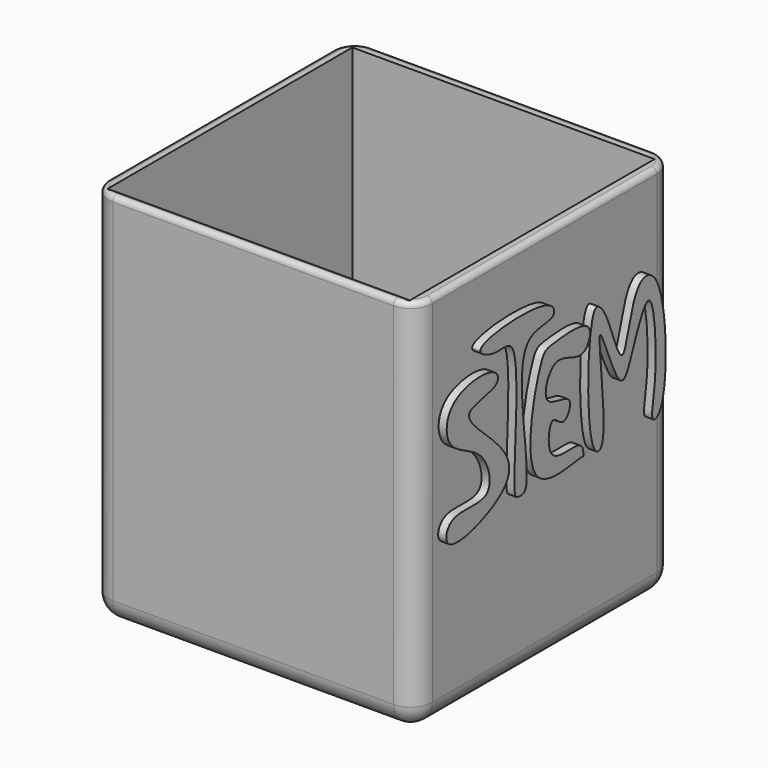
from build123d import *

# Parameters (mm, degrees)
F0_W        = 76.2
F0_H        = 76.2
F1_DEPTH    = 88.9
F2_T        = -2.54
F3_R        = 5.08
F4_R        = 1.27
F5_T1_DEPTH = 71.12
F6_R        = 5.08
F8_DEPTH    = 1.905
F10_DEPTH   = 1.905
F12_DEPTH   = 1.905


# Not quite as in the source:
# - a fillet or chamfer that OpenCascade refuses, or shapes differently, is made with other operations: its cross-section is extruded or revolved along the edge and cut away or added


with BuildPart() as f1:
    # F0 (on Top) → F1 (new body)
    with BuildSketch(Plane.XY):
        Rectangle(F0_W, F0_H)
    extrude(amount=-F1_DEPTH)

    # F2
    f2_openings = [f1.faces().sort_by_distance(p)[0] for p in [
        (0, 0, 0),
    ]]
    offset(amount=F2_T, openings=f2_openings)

    # F3
    f3_edges = [f1.edges().sort_by_distance(p)[0] for p in [
        (38.1, 38.1, -44.45),
        (-38.1, 38.1, -44.45),
        (38.1, -38.1, -44.45),
        (-38.1, -38.1, -44.45),
    ]]
    fillet(f3_edges, radius=F3_R)

    # F4
    f4_edges = [f1.edges().sort_by_distance(p)[0] for p in [
        (0, 38.1, 0),
    ]]
    fillet(f4_edges, radius=F4_R)

    # F5: fillet of radius 1.27 on 1 edges, made by hand

    # F5_s2 → F5_t1 (cut)
    with BuildSketch(Plane.YZ.offset(-35.56)):
        with BuildLine():
            ThreePointArc((-36.83, 0), (-35.9319743879, -0.3719743879), (-35.56, -1.27))
            Line((-35.56, -1.27), (-35.56, 0))
            Line((-35.56, 0), (-36.83, 0))
        make_face()
    extrude(amount=F5_T1_DEPTH, mode=Mode.SUBTRACT)

    # F6
    f6_edges = [f1.edges().sort_by_distance(p)[0] for p in [
        (0, -38.1, -88.9),
        (-36.612102, -36.612102, -88.9),
        (36.612102, -36.612102, -88.9),
        (-38.1, 0, -88.9),
        (38.1, 0, -88.9),
        (-36.612102, 36.612102, -88.9),
        (36.612102, 36.612102, -88.9),
        (0, 38.1, -88.9),
    ]]
    fillet(f6_edges, radius=F6_R)


with BuildPart() as f8:
    # F7 (on face) → F8 (new body)
    with BuildSketch(Plane.YZ.offset(38.1)):
        with BuildLine():
            add(Edge.make_bspline(
                [(-17.006078735, -21.4026272297), (-15.8962322568, -22.1380952084), (-15.4425986774, -25.3643620246), (-30.0363187001, -25.3482696676), (-14.9435072905, -36.223189415), (-9.3400033453, -47.4032043895), (-33.013045168, -55.2479526452), (-30.4976979499, -44.3379706459), (-16.5118722798, -48.7838673293), (-19.7908103732, -34.8921321106), (-31.7362766204, -33.1154766319), (-31.5811889142, -20.5936442783), (-19.3819629064, -19.8281871936), (-17.006078735, -21.4026272297)],
                knots=[0, 0, 0, 0, 0.0490952913, 0.1352797639, 0.2422279569, 0.3366327755, 0.4619223519, 0.5262345776, 0.6221933314, 0.7098122158, 0.8088517884, 0.8949001256, 1, 1, 1, 1], degree=3))
        make_face()
    extrude(amount=F8_DEPTH)


with BuildPart() as f8b:
    # F7 (on face) → F8, piece 2 (new body)
    with BuildSketch(Plane.YZ.offset(38.1)):
        with BuildLine():
            add(Edge.make_bspline(
                [(-11.7039000615, -18.7515374273), (-9.29784816, -23.6386816622), (-12.4052967378, -49.5620570181), (-10.1964973647, -49.9353788123), (-4.8196268006, -50.7902677124), (-14.0671805698, -14.9159542243), (1.2256938672, -18.306654789), (-0.0002290339, -11.3743179626), (-27.0387996227, -13.3722527256), (-16.4682647768, -18.4054018331), (-12.730057488, -16.6672185697), (-11.7039000615, -18.7515374273)],
                knots=[0, 0, 0, 0, 0.2015457439, 0.2455951975, 0.3011224365, 0.4999078972, 0.6056569609, 0.6688157617, 0.833306949, 0.9140427263, 1, 1, 1, 1], degree=3))
        make_face()
    extrude(amount=F8_DEPTH)


with BuildPart() as f8c:
    # F7 (on face) → F8, piece 3 (new body)
    with BuildSketch(Plane.YZ.offset(38.1)):
        with BuildLine():
            add(Edge.make_bspline(
                [(-3.2408058178, -24.6655065566), (-5.3489181379, -29.2226148599), (-11.7776280083, -55.1658367452), (8.9494333514, -48.6650860104), (8.9980814907, -49.7811227809), (9.5638461616, -44.5426340155), (-2.4443059355, -48.914143268), (-0.8119915195, -35.3819401572), (3.308189068, -41.8606927474), (7.1824505681, -34.1135956532), (-4.3855243505, -35.7610650543), (0.2750518242, -23.1843955656), (9.1205419756, -30.7866196324), (13.3054506136, -20.8090576334), (-0.8086393145, -22.445813809), (-2.3824062398, -22.809903415), (-3.2408058178, -24.6655065566)],
                knots=[0, 0, 0, 0, 0.1371990972, 0.2385881701, 0.2492737426, 0.2948349876, 0.3769797762, 0.4516194813, 0.5041770491, 0.5608730736, 0.63505393, 0.7103549993, 0.7896774666, 0.8522330552, 0.9441340739, 1, 1, 1, 1], degree=3))
        make_face()
    extrude(amount=F8_DEPTH)


with BuildPart() as f8d:
    # F7 (on face) → F8, piece 4 (new body)
    with BuildSketch(Plane.YZ.offset(38.1)):
        with BuildLine():
            add(Edge.make_bspline(
                [(12.2578702867, -49.1371005774), (9.6120794936, -44.462427749), (10.2189050013, -18.0613561741), (15.0348603633, -20.9242121889), (17.2316249432, -26.4352493468), (21.3454779936, -38.1139422926), (23.2831913102, -19.0136969953), (33.5246391614, -18.9469005683), (34.3660222173, -48.8631022129), (28.6803082446, -51.0376753454), (29.9570289787, -44.2451592734), (30.7421892953, -36.3654670593), (29.0077281408, -19.6614527112), (23.5307944881, -33.1106469524), (19.8402223214, -43.1296325054), (10.661597006, -12.4582488692), (17.1340584188, -50.5948006336), (12.9981784765, -50.4451021732), (12.2578702867, -49.1371005774)],
                knots=[0, 0, 0, 0, 0.1097534127, 0.1384687295, 0.1933311897, 0.245712941, 0.3189141932, 0.3652292419, 0.4725088547, 0.5062939472, 0.5511851893, 0.6167172321, 0.682835557, 0.7470710185, 0.7965060051, 0.8710684293, 0.9692903345, 1, 1, 1, 1], degree=3))
        make_face()
    extrude(amount=F8_DEPTH)


with BuildPart() as f10:
    # F9 (on face) → F10 (new body)
    with BuildSketch(Plane(origin=(-38.1, 0, 0), x_dir=(0, -1, 0), z_dir=(-1, 0, 0))):
        with BuildLine():
            add(Edge.make_bspline(
                [(18.729981035, -17.2678530216), (16.3288762208, -22.1063473732), (13.8526939321, -37.0180606564), (20.1758040048, -42.1062282851), (20.2078211883, -27.123943743), (28.1645281176, -25.6110096358), (26.4150006448, -41.8335023676), (35.1095596219, -38.4545875902), (29.4793366996, -10.3710164201), (22.8470272161, -12.9205373436), (20.0671258207, -14.5733569485), (18.729981035, -17.2678530216)],
                knots=[0, 0, 0, 0, 0.1684366982, 0.2373892792, 0.3661985221, 0.4399832213, 0.5711037493, 0.6427696468, 0.8303382576, 0.9061997413, 1, 1, 1, 1], degree=3))
        make_face()
        with BuildLine():
            add(Edge.make_bspline(
                [(23.3911480755, -17.2678530216), (22.2090270683, -18.8787588205), (18.5254059552, -23.8735365293), (31.575254183, -26.0675426018), (25.5678997596, -14.2876797507), (24.1422976777, -16.2442427121), (23.3911480755, -17.2678530216)],
                knots=[0, 0, 0, 0, 0.2597555321, 0.5339073663, 0.8349447616, 1, 1, 1, 1], degree=3))
        make_face(mode=Mode.SUBTRACT)
    extrude(amount=F10_DEPTH)


with BuildPart() as f10b:
    # F9 (on face) → F10, piece 2 (new body)
    with BuildSketch(Plane(origin=(-38.1, 0, 0), x_dir=(0, -1, 0), z_dir=(-1, 0, 0))):
        with BuildLine():
            add(Edge.make_bspline(
                [(-31.7203216255, -38.2431149483), (-34.0674151494, -34.7750170896), (-32.3858637197, -15.0543270552), (-29.4641552559, -12.1316251435), (-26.1151954526, -14.0648863336), (-24.5359219279, -22.7678342479), (-17.5507965601, -8.3933242801), (-14.2096307617, -23.7393936366), (-12.3569969127, -38.1214494925), (-19.5053526604, -37.8240881189), (-17.518587556, -17.0915841757), (-23.921786835, -26.2461017733), (-26.7773202902, -18.1643675942), (-31.8255224825, -20.5042513636), (-26.7275801266, -39.2828888495), (-30.9498201783, -39.3816185451), (-31.7203216255, -38.2431149483)],
                knots=[0, 0, 0, 0, 0.1264965791, 0.1746536345, 0.2222035029, 0.2819136291, 0.3559912588, 0.4411898483, 0.540527599, 0.586003567, 0.6878824134, 0.7414626341, 0.8046871099, 0.8481554365, 0.9584738331, 1, 1, 1, 1], degree=3))
        make_face()
    extrude(amount=F10_DEPTH)


with BuildPart() as f10c:
    # F9 (on face) → F10, piece 3 (new body)
    with BuildSketch(Plane(origin=(-38.1, 0, 0), x_dir=(0, -1, 0), z_dir=(-1, 0, 0))):
        with BuildLine():
            add(Edge.make_bspline(
                [(-2.3823736701, -12.195404619), (-1.216559849, -13.0865506225), (0.219342845, -18.2004485051), (-14.6564422611, -16.6011871775), (-1.4186215049, -26.2016034963), (1.5509247504, -34.9684130194), (-12.5233109703, -39.7014159627), (-12.187947555, -30.3108091322), (-4.7373941749, -34.9526649483), (-1.7898161761, -28.8944513906), (-10.2531806511, -26.4047438403), (-14.9076380328, -17.8309533638), (-8.2443280126, -12.549616749), (-3.7278272132, -11.1669423327), (-2.3823736701, -12.195404619)],
                knots=[0, 0, 0, 0, 0.0653739768, 0.1558530699, 0.25991991, 0.3496907913, 0.4517496681, 0.517929379, 0.5969155501, 0.6579949921, 0.7461226973, 0.8374250158, 0.9245525768, 1, 1, 1, 1], degree=3))
        make_face()
    extrude(amount=F10_DEPTH)


with BuildPart() as f10d:
    # F9 (on face) → F10, piece 4 (new body)
    with BuildSketch(Plane(origin=(-38.1, 0, 0), x_dir=(0, -1, 0), z_dir=(-1, 0, 0))):
        with BuildLine():
            add(Edge.make_bspline(
                [(7.7625256963, -12.7437766641), (10.5878979737, -11.8918596821), (15.9736386594, -11.1283338087), (17.9520763273, -18.5732331848), (10.1291845291, -16.5265013232), (2.81880147, -16.646405065), (8.9578108306, -24.7950797214), (13.5983072337, -24.2793818838), (13.1768109629, -30.7839532421), (13.0935829697, -37.9450254764), (2.2909477426, -38.2315890102), (2.211065388, -30.8134702211), (11.2499244846, -36.9351549181), (12.2800234762, -25.5065623189), (1.1072148447, -25.529426316), (-0.0164683771, -16.0605275078), (4.9157806378, -13.6021380483), (7.7625256963, -12.7437766641)],
                knots=[0, 0, 0, 0, 0.074603046, 0.129278223, 0.1983417355, 0.2578970265, 0.3300778397, 0.3821748247, 0.4445909066, 0.5123277352, 0.5882508891, 0.6381131094, 0.7075409187, 0.7746168256, 0.8551699338, 0.9248326126, 1, 1, 1, 1], degree=3))
        make_face()
    extrude(amount=F10_DEPTH)


with BuildPart() as f12:
    # F11 (on face) → F12 (new body)
    with BuildSketch(Plane(origin=(-38.1, 0, 0), x_dir=(0, -1, 0), z_dir=(-1, 0, 0))):
        with BuildLine():
            add(Edge.make_bspline(
                [(-30.9840403497, -47.7236583829), (-31.8317429347, -48.6513788982), (-32.369154146, -52.426349637), (-28.4936223821, -53.1004610288), (-24.4803978842, -50.8492623457), (-18.9442255446, -50.622456444), (-14.9867964601, -63.1126035526), (-24.0198632022, -67.9176610446), (-29.360230968, -70.7545759063), (-30.2857783885, -77.8244348984), (-22.1868123711, -79.2665135472), (-7.5360801039, -81.7965024049), (-9.6828572252, -70.1801908109), (-18.2317103735, -75.7135518237), (-23.6641263939, -70.992342207), (-16.5720696684, -69.6709266763), (-11.7919330948, -63.4213737086), (-9.7269325669, -55.3990917503), (-16.9559869984, -47.9919846055), (-26.5602242763, -47.2846720141), (-30.1363378171, -46.7959379249), (-30.9840403497, -47.7236583829)],
                knots=[0, 0, 0, 0, 0.0417904117, 0.0770559104, 0.1216636096, 0.1654103171, 0.2316509997, 0.2936289169, 0.3444235698, 0.3905703049, 0.4478995129, 0.5205301314, 0.5702275553, 0.6285797592, 0.6703701649, 0.7159558753, 0.7747392099, 0.831143322, 0.8935520037, 0.9582095909, 1, 1, 1, 1], degree=3))
        make_face()
    extrude(amount=F12_DEPTH)


with BuildPart() as f12b:
    # F11 (on face) → F12, piece 2 (new body)
    with BuildSketch(Plane(origin=(-38.1, 0, 0), x_dir=(0, -1, 0), z_dir=(-1, 0, 0))):
        with BuildLine():
            add(Edge.make_bspline(
                [(-5.2902940661, -49.1918735206), (-7.6724126843, -51.7298746523), (-8.4846599399, -60.9261013303), (-6.1500265929, -72.3810453976), (-5.3937489795, -79.8006460607), (0.4329463474, -79.7930686418), (5.8220317333, -75.7861283646), (7.130082655, -66.1435086272), (7.9053054648, -56.5330278971), (3.5631944055, -45.5099959639), (-3.3544538832, -47.1293546614), (-5.2902940661, -49.1918735206)],
                knots=[0, 0, 0, 0, 0.1304379489, 0.2659408379, 0.3606735679, 0.4406743328, 0.5354511622, 0.6516576597, 0.7740918185, 0.8939989718, 1, 1, 1, 1], degree=3))
        make_face()
        with BuildLine():
            add(Edge.make_bspline(
                [(-2.720918972, -53.780041635), (-5.5375122273, -56.3288301104), (-5.2463531132, -69.5647574712), (-0.0282260089, -76.768567892), (3.0732985649, -70.8732517702), (3.4583138112, -63.4813521349), (5.3038115549, -53.3263412627), (-1.0011394894, -52.2237806742), (-2.720918972, -53.780041635)],
                knots=[0, 0, 0, 0, 0.2355307835, 0.3871046197, 0.50907961, 0.6802676131, 0.8561876095, 1, 1, 1, 1], degree=3))
        make_face(mode=Mode.SUBTRACT)
    extrude(amount=F12_DEPTH)


with BuildPart() as f12c:
    # F11 (on face) → F12, piece 3 (new body)
    with BuildSketch(Plane(origin=(-38.1, 0, 0), x_dir=(0, -1, 0), z_dir=(-1, 0, 0))):
        with BuildLine():
            add(Edge.make_bspline(
                [(8.8412659243, -47.9071848094), (7.8423684684, -50.4820898852), (10.0225542445, -56.9386455313), (10.5284500298, -71.5946922622), (10.5761019849, -78.8038055267), (16.1652146356, -78.1916485119), (14.6287566698, -71.9375608897), (15.1678872247, -62.1865435108), (15.2841989518, -52.0376036489), (13.6549490246, -42.0063241767), (9.5999487799, -45.9514922363), (8.8412659243, -47.9071848094)],
                knots=[0, 0, 0, 0, 0.1207531338, 0.278909395, 0.3760665006, 0.4473700277, 0.5385945988, 0.6664077003, 0.8021197159, 0.9082855484, 1, 1, 1, 1], degree=3))
        make_face()
    extrude(amount=F12_DEPTH)


with BuildPart() as f12d:
    # F11 (on face) → F12, piece 4 (new body)
    with BuildSketch(Plane(origin=(-38.1, 0, 0), x_dir=(0, -1, 0), z_dir=(-1, 0, 0))):
        with BuildLine():
            add(Edge.make_bspline(
                [(29.3962638825, -43.8695959747), (30.9178101008, -44.3201316087), (33.2498897704, -48.7458561761), (20.6420009658, -49.6299101638), (21.7243583456, -54.4914692505), (18.674247486, -64.5456663026), (31.4308450296, -56.0037495915), (34.3443937584, -82.4640817582), (16.6586135952, -76.8097796133), (16.3018919599, -67.7401268255), (15.957341283, -50.5065996498), (26.5953513973, -43.0402351132), (29.3962638825, -43.8695959747)],
                knots=[0, 0, 0, 0, 0.0632815407, 0.1637191825, 0.2328855768, 0.3175397085, 0.4079105517, 0.540679911, 0.6512944269, 0.7472175982, 0.8835092518, 1, 1, 1, 1], degree=3))
        make_face()
        with BuildLine():
            add(Edge.make_bspline(
                [(20.0218129903, -66.4277374744), (18.948982151, -68.1049661118), (18.4289731159, -73.2184293143), (24.3703292393, -75.9620006436), (28.7748679672, -75.0673120925), (30.6362931983, -67.6768277604), (24.3381413322, -63.3273288663), (20.9633959548, -64.9556974709), (20.0218129903, -66.4277374744)],
                knots=[0, 0, 0, 0, 0.1768255767, 0.3465946998, 0.4870427311, 0.665047847, 0.8448068935, 1, 1, 1, 1], degree=3))
        make_face(mode=Mode.SUBTRACT)
    extrude(amount=F12_DEPTH)


solid = Compound([f1.part, f8.part, f8b.part, f8c.part, f8d.part, f10.part, f10b.part, f10c.part, f10d.part, f12.part, f12b.part, f12c.part, f12d.part])
